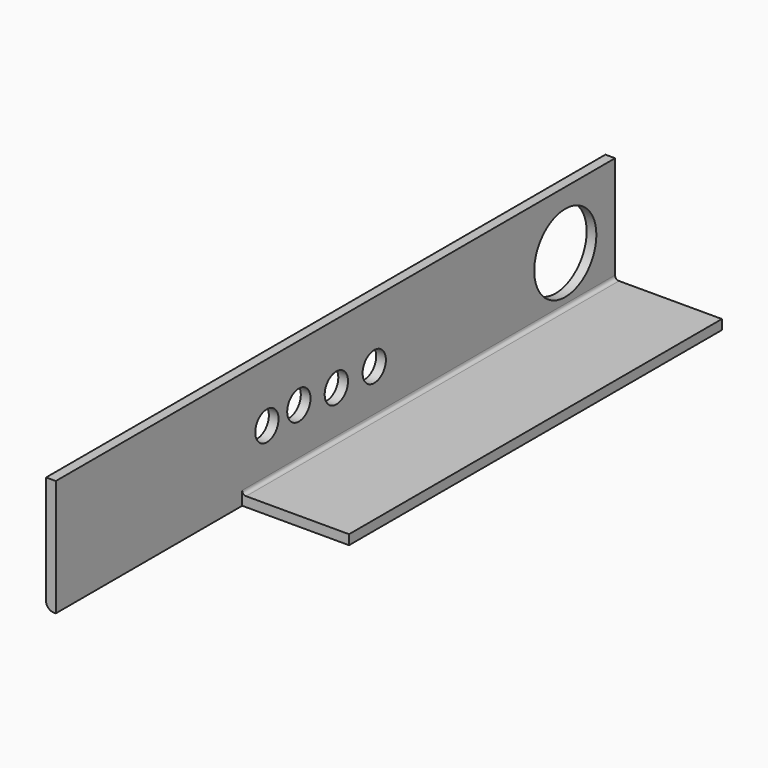
from build123d import *

# Parameters (mm, degrees)
F0_W        = 76.2
F0_H        = 304.8
F1_DEPTH    = 6.35
F2_W        = 457.2
F2_H        = 76.2
F3_DEPTH    = 6.35
F4_R        = 5.08
F5_T1_DEPTH = 304.8
F6_R        = 9.525
F7_DEPTH    = 25.4
F8_R        = 9.525
F9_DEPTH    = 25.4
F10_R       = 9.525
F11_DEPTH   = 25.4
F12_R       = 9.525
F13_DEPTH   = 25.4
F14_R       = 25.4
F15_DEPTH   = 25.4


# Not quite as in the source:
# - a fillet or chamfer that OpenCascade refuses, or shapes differently, is made with other operations: its cross-section is extruded or revolved along the edge and cut away or added


with BuildPart() as f1:
    # F0 (on Top) → F1 (new body)
    with BuildSketch(Plane.XY):
        with Locations((38.1, -152.4)):
            Rectangle(F0_W, F0_H)
    extrude(amount=F1_DEPTH)

    # F2 (on Right) → F3 (join)
    with BuildSketch(Plane.YZ):
        with Locations((-228.6, 38.1)):
            Rectangle(F2_W, F2_H)
    extrude(amount=F3_DEPTH)

    # F4
    f4_edges = [f1.edges().sort_by_distance(p)[0] for p in [
        (0, -228.6, 0),
    ]]
    fillet(f4_edges, radius=F4_R)

    # F5: fillet of radius 2.54 on 1 edges, made by hand

    # F5_s2 → F5_t1 (join)
    with BuildSketch(Plane.XZ):
        with BuildLine():
            add(Edge.make_bspline(
                [(8.89, 6.35), (6.35, 6.35), (6.35, 8.89)],
                knots=[0, 0, 0, 1, 1, 1], degree=2, weights=[1, 1, 1]))
            Line((6.35, 8.89), (6.35, 6.35))
            Line((6.35, 6.35), (8.89, 6.35))
        make_face()
    extrude(amount=F5_T1_DEPTH)

    # F6 (on face) → F7 (cut)
    with BuildSketch(Plane.YZ.offset(6.35)):
        with Locations((-284.6438884735, 37.907961756)):
            Circle(F6_R)
    extrude(amount=-F7_DEPTH, mode=Mode.SUBTRACT)

    # F8 (on face) → F9 (cut)
    with BuildSketch(Plane.YZ.offset(6.35)):
        with Locations((-258.5102617741, 39.1981378198)):
            Circle(F8_R)
    extrude(amount=-F9_DEPTH, mode=Mode.SUBTRACT)

    # F10 (on face) → F11 (cut)
    with BuildSketch(Plane.YZ.offset(6.35)):
        with Locations((-227.8595268726, 36.6169922054)):
            Circle(F10_R)
    extrude(amount=-F11_DEPTH, mode=Mode.SUBTRACT)

    # F12 (on face) → F13 (cut)
    with BuildSketch(Plane.YZ.offset(6.35)):
        with Locations((-196.8858391047, 36.2943448126)):
            Circle(F12_R)
    extrude(amount=-F13_DEPTH, mode=Mode.SUBTRACT)

    # F14 (on face) → F15 (cut)
    with BuildSketch(Plane.YZ.offset(6.35)):
        with Locations((-40.7262966037, 38.2302068174)):
            Circle(F14_R)
    extrude(amount=-F15_DEPTH, mode=Mode.SUBTRACT)


solid = f1.part
